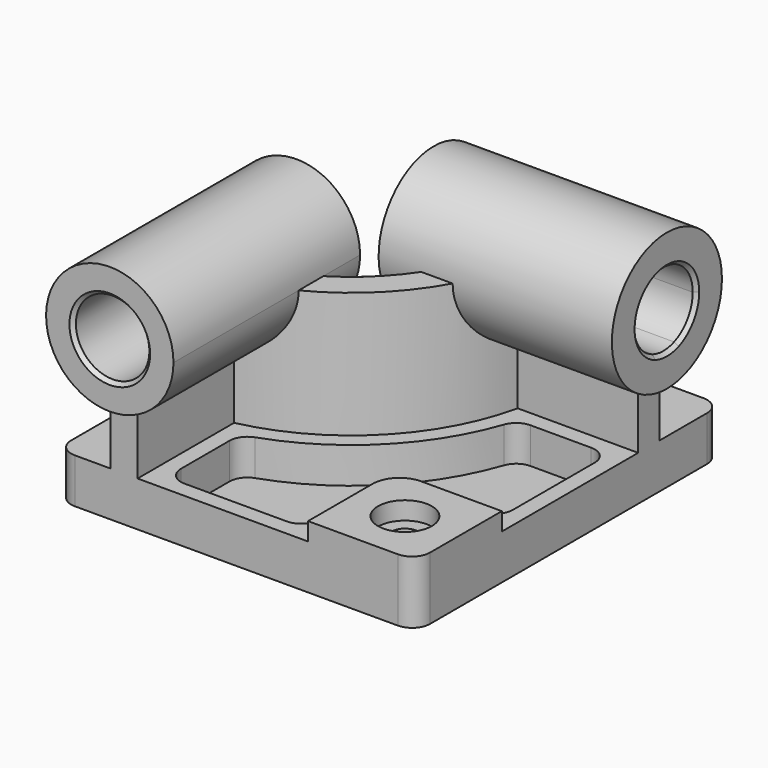
from build123d import *

# Parameters (mm, degrees)
F0_W            = 200
F0_H            = 213
F1_DEPTH        = 95
F2_W            = 60
F2_H            = 60
F3_DEPTH        = 60
F4_DEPTH        = 90
F5_DEPTH        = 70
F6_DEPTH        = 70
F9_DEPTH        = 10
F9_DEPTH_BACK   = 120
F10_R           = 20.5
F11_DEPTH       = 223.001
F12_DEPTH       = 10
F12_DEPTH_BACK  = 120
F13_DEPTH       = 200.001
F13_DEPTH_BACK  = 10.001
F15_D           = 15
F15_CBORE_D     = 30
F15_CBORE_DEPTH = 10
F16_R           = 10
F17_R           = 10
F18_R           = 15
F19_SIZE        = 2


with BuildPart() as f1:
    # F0 (on Top) → F1 (new body)
    with BuildSketch(Plane.XY):
        Rectangle(F0_W, F0_H)
    extrude(amount=F1_DEPTH)

    # F2 (on face) → F3 (cut)
    with BuildSketch(Plane.XY.offset(95)):
        with Locations((70, -76.5)):
            Rectangle(F2_W, F2_H)
    extrude(amount=-F3_DEPTH, mode=Mode.SUBTRACT)

    # F2 (on face) → F4 (cut)
    with BuildSketch(Plane.XY.offset(95)):
        with BuildLine():
            Line((-46, -46.333278), (-46, -97.5))
            Line((-46, -97.5), (31, -97.5))
            Line((31, -97.5), (31, -37.5))
            Line((31, -37.5), (91, -37.5))
            Line((91, -37.5), (91, 39.5))
            Line((91, 39.5), (39.833278, 39.5))
            ThreePointArc((39.833278, 39.5), (8.13768, -14.63768), (-46, -46.333278))
        make_face()
    extrude(amount=-F4_DEPTH, mode=Mode.SUBTRACT)

    # F2 (on face) → F5 (cut)
    with BuildSketch(Plane.XY.offset(95)):
        with BuildLine():
            Line((-55, -39.306845), (-55, -106.5))
            Line((-55, -106.5), (40, -106.5))
            Line((40, -106.5), (40, -46.5))
            Line((40, -46.5), (100, -46.5))
            Line((100, -46.5), (100, 48.5))
            Line((100, 48.5), (32.806845, 48.5))
            ThreePointArc((32.806845, 48.5), (1.773719, -8.273719), (-55, -39.306845))
        make_face()
        with BuildLine():
            Line((31, -97.5), (-46, -97.5))
            Line((-46, -97.5), (-46, -46.333278))
            ThreePointArc((-46, -46.333278), (8.13768, -14.63768), (39.833278, 39.5))
            Line((39.833278, 39.5), (91, 39.5))
            Line((91, 39.5), (91, -37.5))
            Line((91, -37.5), (31, -37.5))
            Line((31, -37.5), (31, -97.5))
        make_face(mode=Mode.SUBTRACT)
    extrude(amount=-F5_DEPTH, mode=Mode.SUBTRACT)

    # F2 (on face) → F6 (cut)
    with BuildSketch(Plane.XY.offset(95)):
        with BuildLine():
            Line((-100, -106.5), (-70, -106.5))
            Line((-70, -106.5), (-70, -26.5))
            ThreePointArc((-70, -26.5), (-8.832882, 2.332882), (20, 63.5))
            Line((20, 63.5), (100, 63.5))
            Line((100, 63.5), (100, 106.5))
            Line((100, 106.5), (-100, 106.5))
            Line((-100, 106.5), (-100, -106.5))
        make_face()
    extrude(amount=-F6_DEPTH, mode=Mode.SUBTRACT)

    # F7 (on face) → F9 (join, two sides)
    with BuildSketch(Plane.XZ.offset(106.5)) as f9_sk:
        with BuildLine():
            ThreePointArc((-42, 95), (-74.043396, 111.941074), (-70, 75.921216))
            Line((-70, 75.921216), (-70, 95))
            Line((-70, 95), (-55, 95))
            Line((-55, 95), (-55, 75.921216))
            ThreePointArc((-55, 75.921216), (-45.558926, 83.456604), (-42, 95))
        make_face()
        with BuildLine():
            Line((-70, 95), (-70, 75.921216))
            ThreePointArc((-70, 75.921216), (-62.5, 74.5), (-55, 75.921216))
            Line((-55, 75.921216), (-55, 95))
            Line((-55, 95), (-70, 95))
        make_face()
        with BuildLine():
            ThreePointArc((-55, 60.301297), (-34.87302, 72.706503), (-27, 95))
            ThreePointArc((-27, 95), (-84.793497, 122.62698), (-70, 60.301297))
            Line((-70, 60.301297), (-70, 75.921216))
            ThreePointArc((-70, 75.921216), (-74.043396, 111.941074), (-42, 95))
            ThreePointArc((-42, 95), (-45.558926, 83.456604), (-55, 75.921216))
            Line((-55, 75.921216), (-55, 60.301297))
        make_face()
        with BuildLine():
            Line((-70, 75.921216), (-70, 60.301297))
            ThreePointArc((-70, 60.301297), (-62.5, 59.5), (-55, 60.301297))
            Line((-55, 60.301297), (-55, 75.921216))
            ThreePointArc((-55, 75.921216), (-62.5, 74.5), (-70, 75.921216))
        make_face()
    extrude(amount=F9_DEPTH)
    extrude(f9_sk.sketch, amount=-F9_DEPTH_BACK)

    # F10 (on face) → F11 (cut, through all)
    with BuildSketch(Plane.XZ.offset(116.5)):
        with Locations((-62.5, 95)):
            Circle(F10_R)
    extrude(amount=-F11_DEPTH, mode=Mode.SUBTRACT)

    # F8 (on face) → F12 (join, two sides)
    with BuildSketch(Plane.YZ.offset(100)) as f12_sk:
        with BuildLine():
            ThreePointArc((76.5, 95), (44.456604, 111.941074), (48.5, 75.921216))
            Line((48.5, 75.921216), (48.5, 95))
            Line((48.5, 95), (63.5, 95))
            Line((63.5, 95), (63.5, 75.921216))
            ThreePointArc((63.5, 75.921216), (72.941074, 83.456604), (76.5, 95))
        make_face()
        with BuildLine():
            ThreePointArc((63.5, 57.407861), (85.638795, 70.690317), (94.333, 95))
            ThreePointArc((94.333, 95), (31.690317, 124.638795), (48.5, 57.407861))
            Line((48.5, 57.407861), (48.5, 75.921216))
            ThreePointArc((48.5, 75.921216), (44.456604, 111.941074), (76.5, 95))
            ThreePointArc((76.5, 95), (72.941074, 83.456604), (63.5, 75.921216))
            Line((63.5, 75.921216), (63.5, 57.407861))
        make_face()
        with BuildLine():
            Line((48.5, 95), (48.5, 75.921216))
            ThreePointArc((48.5, 75.921216), (56, 74.5), (63.5, 75.921216))
            Line((63.5, 75.921216), (63.5, 95))
            Line((63.5, 95), (48.5, 95))
        make_face()
        with BuildLine():
            Line((48.5, 75.921216), (48.5, 57.407861))
            ThreePointArc((48.5, 57.407861), (56, 56.667), (63.5, 57.407861))
            Line((63.5, 57.407861), (63.5, 75.921216))
            ThreePointArc((63.5, 75.921216), (56, 74.5), (48.5, 75.921216))
        make_face()
    extrude(amount=F12_DEPTH)
    extrude(f12_sk.sketch, amount=-F12_DEPTH_BACK)

    # F8 (on face) → F13 (cut, two sides)
    with BuildSketch(Plane.YZ.offset(100)) as f13_sk:
        with BuildLine():
            ThreePointArc((76.5, 95), (44.456604, 111.941074), (48.5, 75.921216))
            Line((48.5, 75.921216), (48.5, 95))
            Line((48.5, 95), (63.5, 95))
            Line((63.5, 95), (63.5, 75.921216))
            ThreePointArc((63.5, 75.921216), (72.941074, 83.456604), (76.5, 95))
        make_face()
        with BuildLine():
            Line((48.5, 95), (48.5, 75.921216))
            ThreePointArc((48.5, 75.921216), (56, 74.5), (63.5, 75.921216))
            Line((63.5, 75.921216), (63.5, 95))
            Line((63.5, 95), (48.5, 95))
        make_face()
    extrude(amount=-F13_DEPTH, mode=Mode.SUBTRACT)
    extrude(f13_sk.sketch, amount=F13_DEPTH_BACK, mode=Mode.SUBTRACT)

    # F15 (through all)
    with Locations(Plane.XY.offset(35)):
        with Locations((70, -76.5)):
            CounterBoreHole(F15_D / 2, F15_CBORE_D / 2, F15_CBORE_DEPTH)

    # F16
    f16_edges = [f1.edges().sort_by_distance(p)[0] for p in [
        (-100, 106.5, 12.5),
        (100, 106.5, 12.5),
        (100, -106.5, 17.5),
        (-100, -106.5, 12.5),
    ]]
    fillet(f16_edges, radius=F16_R)

    # F17
    f17_edges = [f1.edges().sort_by_distance(p)[0] for p in [
        (39.833278, 39.5, 15),
        (91, 39.5, 15),
        (91, -37.5, 15),
        (-46, -46.333278, 15),
        (-46, -97.5, 15),
        (31, -97.5, 15),
    ]]
    fillet(f17_edges, radius=F17_R)

    # F18
    f18_edges = [f1.edges().sort_by_distance(p)[0] for p in [
        (31, -37.5, 15),
        (40, -46.5, 30),
    ]]
    fillet(f18_edges, radius=F18_R)

    # F19
    f19_edges = [f1.edges().sort_by_distance(p)[0] for p in [
        (-83, -116.5, 95),
        (-83, 13.5, 95),
        (-20, 35.5, 95),
        (110, 35.5, 95),
    ]]
    chamfer(f19_edges, length=F19_SIZE)


solid = f1.part
